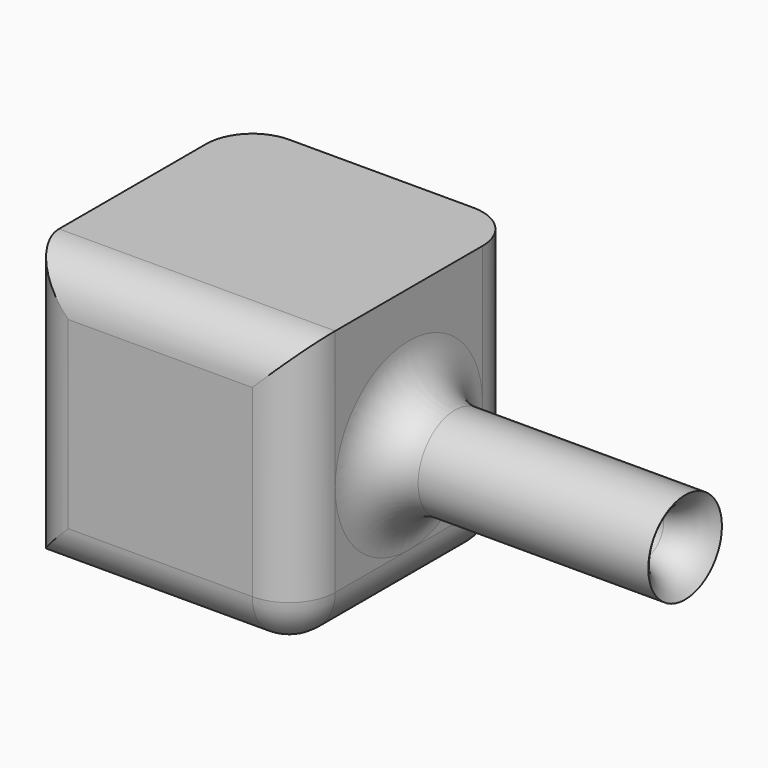
from build123d import *

# Parameters (mm, degrees)
F0_W         = 30
F0_H         = 30
F1_DEPTH     = 30
F2_R         = 5
F3_DEPTH     = 30
F4_R         = 2.5
F5_DEPTH     = 60.001
F6_T3_DEPTH  = 20
F6_T5_DEPTH  = 37.5
F6_T7_DEPTH  = 55
F6_T9_DEPTH  = 55
F6_T11_DEPTH = 37.5
F6_S15_W     = 5.1
F6_S15_H     = 5.1
F6_T16_DEPTH = 5.1
F6_S21_W     = 5.1
F6_S21_H     = 5.1
F6_T22_DEPTH = 5.1


# Not quite as in the source:
# - a fillet or chamfer that OpenCascade refuses, or shapes differently, is made with other operations: its cross-section is extruded or revolved along the edge and cut away or added


with BuildPart() as f1:
    # F0 (on Right) → F1 (new body)
    with BuildSketch(Plane.YZ):
        Rectangle(F0_W, F0_H)
    extrude(amount=F1_DEPTH)

    # F2 (on face) → F3 (join)
    with BuildSketch(Plane.YZ.offset(30)):
        Circle(F2_R)
    extrude(amount=F3_DEPTH)

    # F4 (on face) → F5 (cut, through all)
    with BuildSketch(Plane.YZ.offset(60)):
        Circle(F4_R)
    extrude(amount=-F5_DEPTH, mode=Mode.SUBTRACT)

    # F6: fillet of radius 5 on 11 edges, made by hand

    # F6_s1 → F6_t2 (revolve)
    with BuildSketch(Plane.XY):
        with BuildLine():
            ThreePointArc((30, 10), (31.4644660941, 6.4644660941), (35, 5))
            Line((35, 5), (30, 5))
            Line((30, 5), (30, 10))
        make_face()
    revolve(axis=Axis((30, 0, 0), (1, 0, 0)))

    # F6_s4 → F6_t3 (cut)
    with BuildSketch(Plane.XZ.offset(-10)):
        with BuildLine():
            ThreePointArc((25, -15), (28.5355339059, -13.5355339059), (30, -10))
            Line((30, -10), (30, -15))
            Line((30, -15), (25, -15))
        make_face()
    extrude(amount=F6_T3_DEPTH, mode=Mode.SUBTRACT)

    # F6_s6 → F6_t5 (cut)
    with BuildSketch(Plane.YZ.offset(-12.5)):
        with BuildLine():
            ThreePointArc((15, -10), (13.5355339059, -13.5355339059), (10, -15))
            Line((10, -15), (15, -15))
            Line((15, -15), (15, -10))
        make_face()
        with BuildLine():
            ThreePointArc((-10, -15), (-13.5355339059, -13.5355339059), (-15, -10))
            Line((-15, -10), (-15, -15))
            Line((-15, -15), (-10, -15))
        make_face()
    extrude(amount=F6_T5_DEPTH, mode=Mode.SUBTRACT)

    # F6_s8 → F6_t7 (cut)
    with BuildSketch(Plane.YZ.offset(-12.5)):
        with BuildLine():
            ThreePointArc((-10, 15), (-13.5355339059, 13.5355339059), (-15, 10))
            Line((-15, 10), (-15, 15))
            Line((-15, 15), (-10, 15))
        make_face()
    extrude(amount=F6_T7_DEPTH, mode=Mode.SUBTRACT)

    # F6_s10 → F6_t9 (cut)
    with BuildSketch(Plane.XY.offset(-27.5)):
        with BuildLine():
            ThreePointArc((0, -10), (1.4644660941, -13.5355339059), (5, -15))
            Line((5, -15), (0, -15))
            Line((0, -15), (0, -10))
        make_face()
        with BuildLine():
            ThreePointArc((5, 15), (1.4644660941, 13.5355339059), (0, 10))
            Line((0, 10), (0, 15))
            Line((0, 15), (5, 15))
        make_face()
    extrude(amount=F6_T9_DEPTH, mode=Mode.SUBTRACT)

    # F6_s12 → F6_t11 (cut)
    with BuildSketch(Plane.XY.offset(-10)):
        with BuildLine():
            ThreePointArc((30, -10), (28.5355339059, -13.5355339059), (25, -15))
            Line((25, -15), (30, -15))
            Line((30, -15), (30, -10))
        make_face()
        with BuildLine():
            ThreePointArc((25, 15), (28.5355339059, 13.5355339059), (30, 10))
            Line((30, 10), (30, 15))
            Line((30, 15), (25, 15))
        make_face()
    extrude(amount=F6_T11_DEPTH, mode=Mode.SUBTRACT)


with BuildPart() as f6_tool14:
    # F6_s15 → F6_t16 (new body)
    with BuildSketch(Plane.XY.offset(-10)):
        with Locations((27.55, -12.55)):
            Rectangle(F6_S15_W, F6_S15_H)
    extrude(amount=-F6_T16_DEPTH)

    # F6_s17 → F6_t18 (revolve, cut)
    with BuildSketch(Plane(origin=(25, -10, -10), x_dir=(-0.7071067812, 0.7071067812, 0), z_dir=(-0.7071067812, -0.7071067812, 0))):
        with BuildLine():
            ThreePointArc((0, -5), (5, 0), (0, 5))
            Line((0, 5), (0, -5))
        make_face()
    revolve(axis=Axis((25, -10, -10), (0, 0, -1)), mode=Mode.SUBTRACT)


with BuildPart() as f1_1:
    add(f1.part)

    # F6_t13: cut F6_tool14
    add(f6_tool14.part, mode=Mode.SUBTRACT)


with BuildPart() as f6_tool20:
    # F6_s21 → F6_t22 (new body)
    with BuildSketch(Plane.XZ.offset(-10)):
        with Locations((27.55, -12.55)):
            Rectangle(F6_S21_W, F6_S21_H)
    extrude(amount=-F6_T22_DEPTH)

    # F6_s23 → F6_t24 (revolve, cut)
    with BuildSketch(Plane(origin=(25, 10, -10), x_dir=(-0.7071067812, 0, 0.7071067812), z_dir=(-0.7071067812, 0, -0.7071067812))):
        with BuildLine():
            ThreePointArc((0, -5), (5, 0), (0, 5))
            Line((0, 5), (0, -5))
        make_face()
    revolve(axis=Axis((25, 10, -10), (0, 1, 0)), mode=Mode.SUBTRACT)


with BuildPart() as f1_2:
    add(f1_1.part)

    # F6_t19: cut F6_tool20
    add(f6_tool20.part, mode=Mode.SUBTRACT)

    # F6_s25 → F6_t26 (revolve, cut)
    with BuildSketch(Plane.XY):
        with BuildLine():
            ThreePointArc((0, 7.5), (1.4644660941, 3.9644660941), (5, 2.5))
            Line((5, 2.5), (0, 2.5))
            Line((0, 2.5), (0, 7.5))
        make_face()
    revolve(axis=Axis((0, 0, 0), (1, 0, 0)), mode=Mode.SUBTRACT)

    # F6_s27 → F6_t28 (revolve, cut)
    with BuildSketch(Plane.XY):
        with BuildLine():
            ThreePointArc((55.6698729811, 2.5), (58.1698729811, 3.1698729811), (60, 5))
            Line((60, 5), (60, 2.5))
            Line((60, 2.5), (55.6698729811, 2.5))
        make_face()
    revolve(axis=Axis((60, 0, 0), (1, 0, 0)), mode=Mode.SUBTRACT)


solid = f1_2.part
